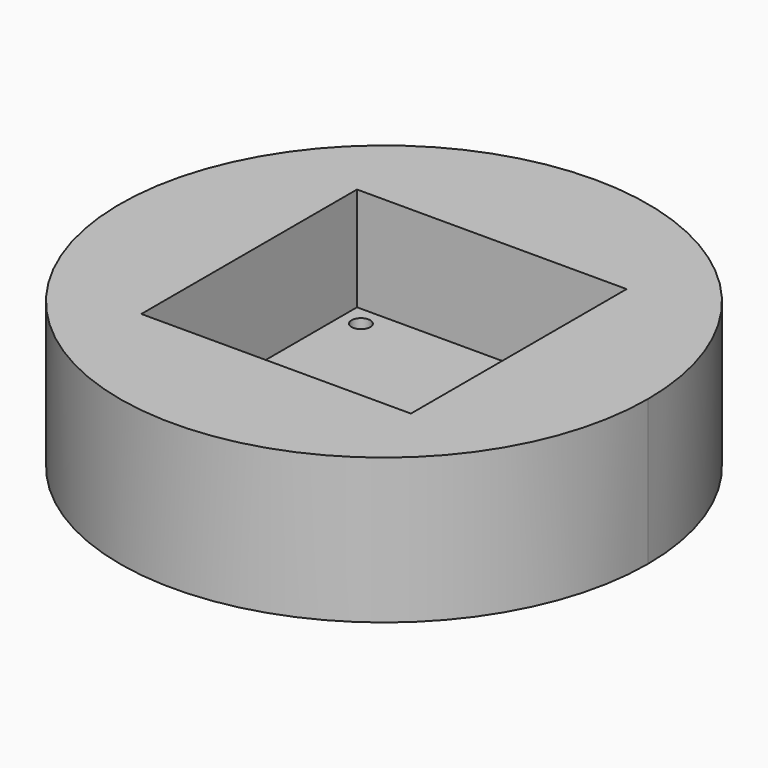
from build123d import *

# Parameters (mm, degrees)
F1_DEPTH = 5.08
F2_W     = 6.35
F2_H     = 33.02
F3_DEPTH = 5.08
F4_DEPTH = 12.7
F5_R     = 1.143
F6_DEPTH = 25.4
F7_W     = 45.72
F7_H     = 45.72
F7_W_2   = 33.02
F7_H_2   = 33.02
F8_DEPTH = 17.78


with BuildPart() as f1:
    # F0 (on Top) → F1 (new body)
    with BuildSketch(Plane.XY):
        Polygon((15.6999393499, 19.6573674963), (-17.3200606501, 19.6573674963), (-17.3200606501, -13.3626325037), (-4.6200606501, -13.3626325037), (-4.6200606501, -8.2826325037), (2.9999393499, -8.2826325037), (2.9999393499, -13.3626325037), (15.6999393499, -13.3626325037), align=None)
    extrude(amount=F1_DEPTH)

    # F2 (on face) → F3 (join)
    with BuildSketch(Plane.XY.offset(5.08)):
        with Locations((18.8749393499, 3.1473674963)):
            Rectangle(F2_W, F2_H)
        Polygon((-17.3200606501, 26.0073674963), (-17.3200606501, 19.6573674963), (15.6999393499, 19.6573674963), (22.0499393499, 19.6573674963), (22.0499393499, 26.0073674963), align=None)
        Polygon((-4.6200606501, -13.3626325037), (-17.3200606501, -13.3626325037), (-17.3200606501, -19.7126325037), (22.0499393499, -19.7126325037), (22.0499393499, -13.3626325037), (15.6999393499, -13.3626325037), (2.9999393499, -13.3626325037), align=None)
        Polygon((-17.3200606501, -13.3626325037), (-17.3200606501, 19.6573674963), (-17.3200606501, 26.0073674963), (-23.6700606501, 26.0073674963), (-23.6700606501, -19.7126325037), (-17.3200606501, -19.7126325037), align=None)
    extrude(amount=-F3_DEPTH)

    # F2 (on face) → F4 (join)
    with BuildSketch(Plane.XY.offset(5.08)):
        Polygon((-17.3200606501, 26.0073674963), (-17.3200606501, 19.6573674963), (15.6999393499, 19.6573674963), (22.0499393499, 19.6573674963), (22.0499393499, 26.0073674963), align=None)
        with Locations((18.8749393499, 3.1473674963)):
            Rectangle(F2_W, F2_H)
        Polygon((-4.6200606501, -13.3626325037), (-17.3200606501, -13.3626325037), (-17.3200606501, -19.7126325037), (22.0499393499, -19.7126325037), (22.0499393499, -13.3626325037), (15.6999393499, -13.3626325037), (2.9999393499, -13.3626325037), align=None)
        Polygon((-17.3200606501, -13.3626325037), (-17.3200606501, 19.6573674963), (-17.3200606501, 26.0073674963), (-23.6700606501, 26.0073674963), (-23.6700606501, -19.7126325037), (-17.3200606501, -19.7126325037), align=None)
    extrude(amount=F4_DEPTH)

    # F5 (on face) → F6 (cut)
    with BuildSketch(Plane.XY.offset(5.08)):
        with Locations((13.2869393499, 17.2443674963)):
            Circle(F5_R)
        with Locations((-14.9070606501, -10.9496325037)):
            Circle(F5_R)
        with Locations((13.2869393499, -10.9496325037)):
            Circle(F5_R)
        with Locations((-14.9070606501, 17.2443674963)):
            Circle(F5_R)
    extrude(amount=-F6_DEPTH, mode=Mode.SUBTRACT)

    # F7 (on face) → F8 (join)
    with BuildSketch(Plane.XY.offset(17.78)):
        with BuildLine():
            ThreePointArc((22.0499393499, -19.7126325037), (29.057968727, -9.224375353), (31.5188613857, 3.1473674963))
            ThreePointArc((31.5188613857, 3.1473674963), (29.057968727, 15.5191103457), (22.0499393499, 26.0073674963))
            Line((22.0499393499, 26.0073674963), (22.0499393499, -19.7126325037))
        make_face()
        with BuildLine():
            Line((-23.6700606501, 26.0073674963), (22.0499393499, 26.0073674963))
            ThreePointArc((22.0499393499, 26.0073674963), (-0.8100606501, 35.4762895322), (-23.6700606501, 26.0073674963))
        make_face()
        with Locations((-0.8100606501, 3.1473674963)):
            Rectangle(F7_W, F7_H)
        with Locations((-0.8100606501, 3.1473674963)):
            Rectangle(F7_W_2, F7_H_2, mode=Mode.SUBTRACT)
        with BuildLine():
            ThreePointArc((-23.6700606501, -19.7126325037), (-0.8100606501, -29.1815545395), (22.0499393499, -19.7126325037))
            Line((22.0499393499, -19.7126325037), (-23.6700606501, -19.7126325037))
        make_face()
        with BuildLine():
            Line((-23.6700606501, -19.7126325037), (-23.6700606501, 26.0073674963))
            ThreePointArc((-23.6700606501, 26.0073674963), (-33.138982686, 3.1473674963), (-23.6700606501, -19.7126325037))
        make_face()
    extrude(amount=-F8_DEPTH)


solid = f1.part
